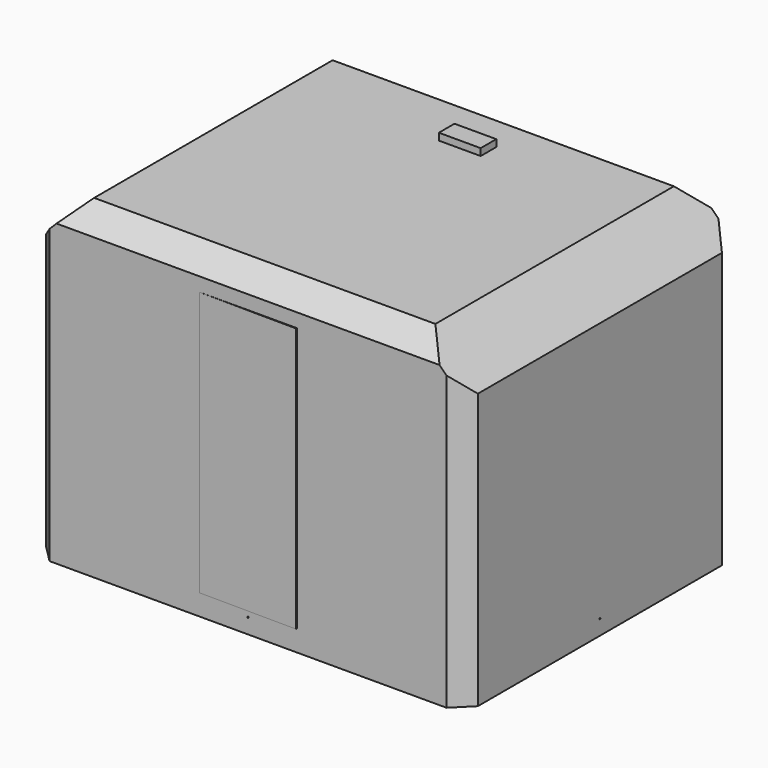
from build123d import *

# Parameters (mm, degrees)
F0_W           = 3100
F0_H           = 2300
F1_DEPTH       = 2440
F2_SIZE        = 325
F3_SIZE        = 325
F4_SIZE        = 125
F5_SIZE        = 125
F6_SIZE        = 125
F7_SIZE        = 125
F8_W           = 1519
F8_H           = 1519
F9_DEPTH       = 108
F10_W          = 400
F10_H          = 200
F10_R          = 7.5
F11_DEPTH      = 1
F12_R          = 5
F13_DEPTH      = 1
F14_DEPTH      = 790.501
F14_DEPTH_BACK = 2309.501
F15_R          = 5
F16_DEPTH      = 460.501
F16_DEPTH_BACK = 1979.501
F17_SIZE       = 150
F18_SIZE       = 150
F19_W          = 1719
F19_H          = 1719
F19_W_2        = 1519
F19_H_2        = 1519
F20_DEPTH      = 15
F21_W          = 700
F21_H          = 1900
F22_DEPTH      = 20
F23_W          = 300
F23_H          = 140
F24_DEPTH      = 50
F26_DEPTH      = 1900


# Not quite as in the source:
# - a feature of the source that left no trace in its solid (it failed there, or was rolled back) is left out


with BuildPart() as f1:
    # F0 (on Front) → F1 (new body)
    with BuildSketch(Plane.XZ):
        Rectangle(F0_W, F0_H)
    extrude(amount=F1_DEPTH)

    # F2
    f2_edges = [f1.edges().sort_by_distance(p)[0] for p in [
        (-1550, -1220, 1150),
    ]]
    chamfer(f2_edges, length=F2_SIZE)

    # F3
    f3_edges = [f1.edges().sort_by_distance(p)[0] for p in [
        (1550, -1220, 1150),
    ]]
    chamfer(f3_edges, length=F3_SIZE)

    # F4
    f4_edges = [f1.edges().sort_by_distance(p)[0] for p in [
        (1550, -2440, -162.5),
    ]]
    chamfer(f4_edges, length=F4_SIZE)

    # F5
    f5_edges = [f1.edges().sort_by_distance(p)[0] for p in [
        (-1550, -2440, -162.5),
    ]]
    chamfer(f5_edges, length=F5_SIZE)

    # F6
    f6_edges = [f1.edges().sort_by_distance(p)[0] for p in [
        (-1550, 0, -162.5),
    ]]
    chamfer(f6_edges, length=F6_SIZE)

    # F7
    f7_edges = [f1.edges().sort_by_distance(p)[0] for p in [
        (1550, 0, -162.5),
    ]]
    chamfer(f7_edges, length=F7_SIZE)

    # F8 (on face) → F9 (cut)
    with BuildSketch(Plane(origin=(0, 0, -1150), x_dir=(1, 0, 0), z_dir=(0, 0, -1))):
        with Locations((0, 1220)):
            Rectangle(F8_W, F8_H)
    extrude(amount=-F9_DEPTH, mode=Mode.SUBTRACT)

    # F10 (on face) → F11 (cut)
    with BuildSketch(Plane(origin=(0, 0, -1042), x_dir=(1, 0, 0), z_dir=(0, 0, -1))):
        with Locations((0, 1769.5)):
            Rectangle(F10_W, F10_H)
        with Locations((0, 1849.5)):
            Circle(F10_R, mode=Mode.SUBTRACT)
        Polygon((601.4287087912, 1174.2050807569), (428.2236280343, 1274.2050807569), (228.2236280343, 927.7949192431), (401.4287087912, 827.7949192431), align=None)
        with Locations((484.1082007155, 1011)):
            Circle(F10_R, mode=Mode.SUBTRACT)
        Polygon((-228.2236280343, 927.7949192431), (-428.2236280343, 1274.2050807569), (-601.4287087912, 1174.2050807569), (-401.4287087912, 827.7949192431), align=None)
        with Locations((-484.1082007155, 1011)):
            Circle(F10_R, mode=Mode.SUBTRACT)
        with Locations((0, 1290.5)):
            Circle(F10_R)
    extrude(amount=-F11_DEPTH, mode=Mode.SUBTRACT)

    # F12 (on face) → F13 (cut)
    with BuildSketch(Plane.YZ.offset(-759.5)):
        with Locations((-1220, -1042)):
            Circle(F12_R)
    extrude(amount=F13_DEPTH, mode=Mode.SUBTRACT)

    # F12 (on face) → F14 (cut, two sides)
    with BuildSketch(Plane.YZ.offset(-759.5)) as f14_sk:
        with Locations((-1220, -1042)):
            Circle(F12_R)
    extrude(amount=-F14_DEPTH, mode=Mode.SUBTRACT)
    extrude(f14_sk.sketch, amount=F14_DEPTH_BACK, mode=Mode.SUBTRACT)

    # F15 (on face) → F16 (cut, two sides)
    with BuildSketch(Plane.XZ.offset(460.5)) as f16_sk:
        with Locations((0, -1042)):
            Circle(F15_R)
    extrude(amount=-F16_DEPTH, mode=Mode.SUBTRACT)
    extrude(f16_sk.sketch, amount=F16_DEPTH_BACK, mode=Mode.SUBTRACT)

    # F17
    f17_edges = [f1.edges().sort_by_distance(p)[0] for p in [
        (0, 0, 1150),
    ]]
    chamfer(f17_edges, length=F17_SIZE)

    # F18
    f18_edges = [f1.edges().sort_by_distance(p)[0] for p in [
        (0, -2440, 1150),
    ]]
    chamfer(f18_edges, length=F18_SIZE)

    # F19 (on face) → F20 (join)
    with BuildSketch(Plane(origin=(0, 0, -1150), x_dir=(1, 0, 0), z_dir=(0, 0, -1))):
        with Locations((0, 1220)):
            Rectangle(F19_W, F19_H)
        with Locations((0, 1220)):
            Rectangle(F19_W_2, F19_H_2, mode=Mode.SUBTRACT)
    extrude(amount=F20_DEPTH)

    # F21 (on face) → F22 (cut)
    with BuildSketch(Plane.XZ.offset(2440)):
        with Locations((0, -50)):
            Rectangle(F21_W, F21_H)
    extrude(amount=-F22_DEPTH, mode=Mode.SUBTRACT)

    # F23 (on face) → F24 (join)
    with BuildSketch(Plane.XY.offset(1150)):
        with Locations((0, -470)):
            Rectangle(F23_W, F23_H)
    extrude(amount=F24_DEPTH)

    # F25 (on face) → F26 (join)
    with BuildSketch(Plane.XY.offset(-1000)):
        Polygon((-350, -2420), (-350.17453071, -2439.9992384613), (349.798815435, -2446.1078133101), (349.9733461449, -2426.1085748489), align=None)
    extrude(amount=F26_DEPTH)


solid = f1.part
